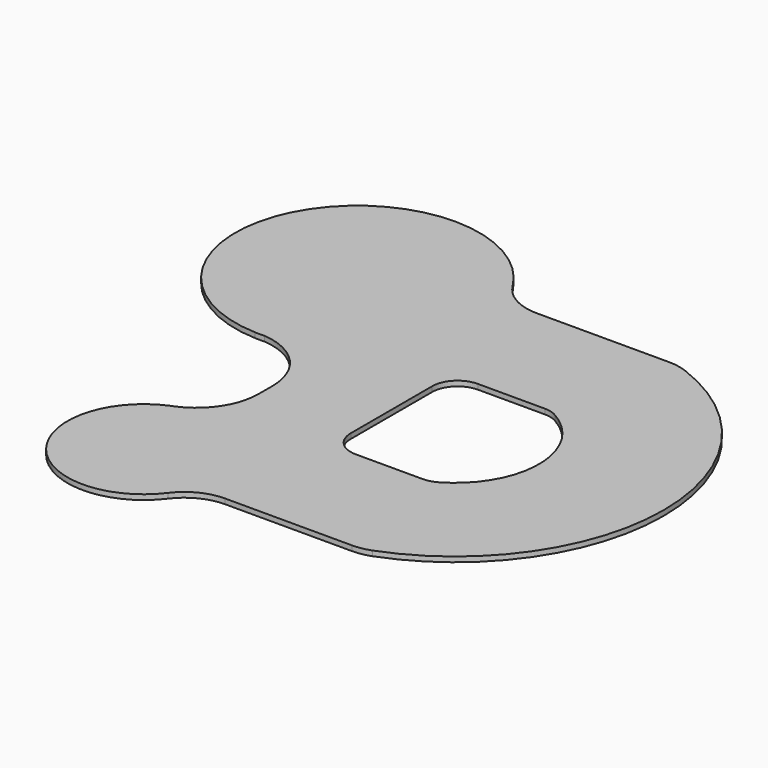
from build123d import *

# Parameters (mm, degrees)
F1_DEPTH = 1
F2_SCALE = 0.5
F3_SCALE = 0.75


# Not quite as in the source:
# - a feature of the source that left no trace in its solid (it failed there, or was rolled back) is left out


with BuildPart() as f1:
    # F0 (on Top) → F1 (new body)
    with BuildSketch(Plane.XY):
        with BuildLine():
            ThreePointArc((28.844410196, 8.0000000124), (23.9936976971, 9.2552536894), (20.3607601383, 12.7058823617))
            ThreePointArc((20.3607601383, 12.7058823617), (-20.765045237, 12.0338230128), (-0.9013340087, -23.9830689655))
            ThreePointArc((-0.9013340087, -23.9830689655), (0, -23.95), (0.9013340087, -23.9830689655))
            ThreePointArc((0.9013340087, -23.9830689655), (9.0104497198, -27.8773184793), (12.3, -36.25))
            Line((12.3, -36.25), (12.3, -39.6172702312))
            ThreePointArc((12.3, -39.6172702312), (10.3056584811, -46.3316877988), (4.9693653218, -50.8687327272))
            ThreePointArc((4.9693653218, -50.8687327272), (4.5085414865, -51.0611792515), (4.0402855379, -51.2347610435))
            ThreePointArc((4.0402855379, -51.2347610435), (-1.7764718202, -74.2905711056), (22, -74))
            ThreePointArc((22, -74), (25.527864045, -71.05572809), (30, -70))
            Line((30, -70), (54.9544511501, -70))
            ThreePointArc((54.9544511501, -70), (56.7505041703, -69.8373875368), (58.4881450694, -69.3548387097))
            ThreePointArc((58.4881450694, -69.3548387097), (85.0000000049, -30.9999999956), (58.488145074, 7.3548387217))
            ThreePointArc((58.488145074, 7.3548387217), (56.7505041744, 7.837387549), (54.9544511536, 8.0000000124))
            Line((54.9544511536, 8.0000000124), (28.844410196, 8.0000000124))
        make_face()
        with BuildLine():
            ThreePointArc((52.1479989309, -16.652173913), (60.5, -31), (52.1479989309, -45.347826087))
            ThreePointArc((52.1479989309, -45.347826087), (50.9557931419, -45.8342078169), (49.6789083458, -46))
            Line((49.6789083458, -46), (36.5, -46))
            ThreePointArc((36.5, -46), (32.9644660941, -44.5355339059), (31.5, -41))
            Line((31.5, -41), (31.5, -21))
            ThreePointArc((31.5, -21), (32.9644660941, -17.4644660941), (36.5, -16))
            Line((36.5, -16), (49.6789083458, -16))
            ThreePointArc((49.6789083458, -16), (50.9557931419, -16.1657921831), (52.1479989309, -16.652173913))
        make_face(mode=Mode.SUBTRACT)
        with BuildLine():
            ThreePointArc((0.9013340087, -23.9830689655), (0, -23.95), (-0.9013340087, -23.9830689655))
            ThreePointArc((-0.9013340087, -23.9830689655), (0, -24), (0.9013340087, -23.9830689655))
        make_face()
        with BuildLine():
            ThreePointArc((4.0402855379, -51.2347610435), (4.5085414865, -51.0611792515), (4.9693653218, -50.8687327272))
            ThreePointArc((4.9693653218, -50.8687327272), (4.501778675, -51.0440133899), (4.0402855379, -51.2347610435))
        make_face()
    extrude(amount=F1_DEPTH)


with BuildPart() as f1_1:
    # F2: moved
    add(f1.part.scale(F2_SCALE))


with BuildPart() as f1_2:
    # F3: moved
    add(f1_1.part.scale(F3_SCALE))


solid = f1_2.part
